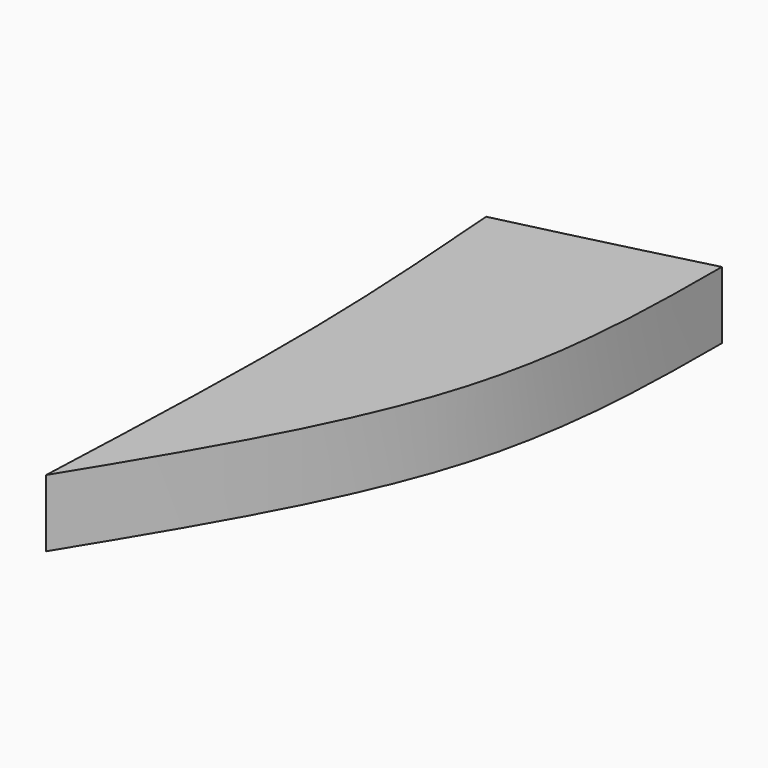
from build123d import *

# Parameters (mm, degrees)
F0_R     = 0.65
F3_DEPTH = 0.9398
F5_DEPTH = 1.016


# Not quite as in the source:
# - a fillet or chamfer that OpenCascade refuses, or shapes differently, is made with other operations: its cross-section is extruded or revolved along the edge and cut away or added
# - a feature names something its author has since deleted; it is built from what else it names


with BuildPart() as f3:
    # F0 (on Top) → F3 (new body)
    with BuildSketch(Plane.XY):
        with Locations((-65.8378056469, 32.2275372886)):
            Circle(F0_R)
    extrude(amount=F3_DEPTH)

    # F4: fillet of radius 0.6 on 1 edges, made by hand

    # F4_s1 → F4_t2 (revolve, cut)
    with BuildSketch(Plane.XZ.offset(-32.2275372886)):
        with BuildLine():
            add(Edge.make_bspline(
                [(-65.1878056469, 0.3398), (-65.1878056469, 0.9398), (-65.7878056469, 0.9398)],
                knots=[0, 0, 0, 1, 1, 1], degree=2, weights=[1, 0.4285714286, 1]))
            Line((-65.7878056469, 0.9398), (-65.1878056469, 0.9398))
            Line((-65.1878056469, 0.9398), (-65.1878056469, 0.3398))
        make_face()
    revolve(axis=Axis((-65.8378056469, 32.2275372886, 0.9398), (0, 0, 1)), mode=Mode.SUBTRACT)


with BuildPart() as f5:
    # F1 (on Top) → F5 (new body)
    with BuildSketch(Plane.XY):
        with BuildLine():
            ThreePointArc((-30.8833700819, -8.5484330949), (-32.3702413361, -8.924628467), (-33.8609412709, -9.285353832))
            add(Edge.make_bspline(
                [(-33.8609412709, -9.285353832), (-33.7752337579, -10.3873432275), (-33.5955934863, -12.7868478548), (-33.721363311, -15.9607901983), (-33.7918073162, -17.6922008293)],
                knots=[0, 0, 0, 0, 0.4545759476, 1, 1, 1, 1], degree=3))
            add(Edge.make_bspline(
                [(-30.8833700819, -8.5484330949), (-30.8858372606, -10.0078512456), (-30.9439518259, -12.998153667), (-32.7959538604, -16.0707410395), (-33.7918073162, -17.6922008293)],
                knots=[0, 0, 0, 0, 0.4714457615, 1, 1, 1, 1], degree=3))
        make_face()
    extrude(amount=-F5_DEPTH)


solid = f5.part
